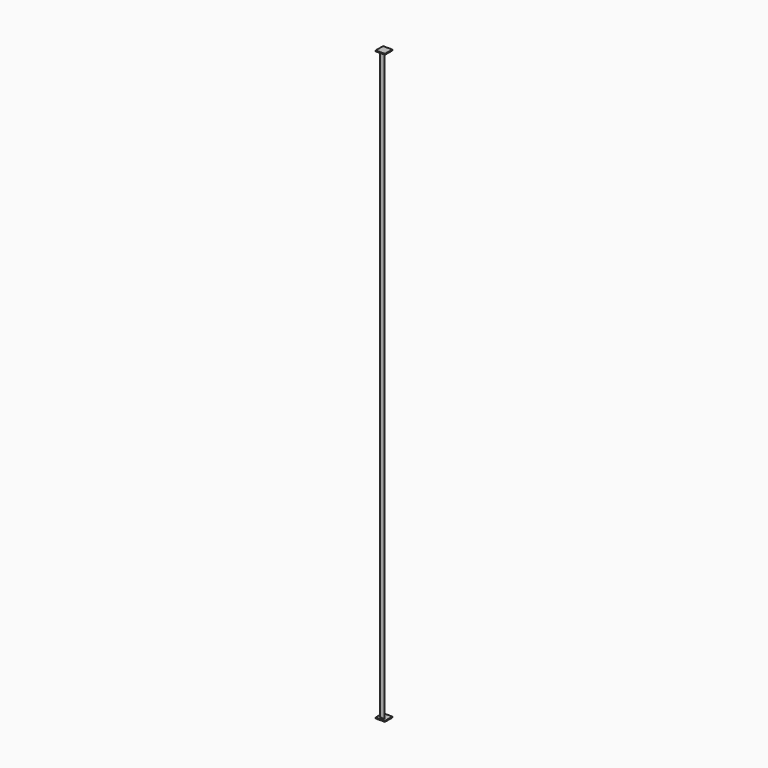
from build123d import *

# Parameters (mm, degrees)
F1_DEPTH = 1894
F2_R     = 2
F3_R     = 1.99999
F4_W     = 30
F4_H     = 30
F5_DEPTH = 3
F6_W     = 30
F6_H     = 30
F7_DEPTH = 3


# Not quite as in the source:
# - a fillet or chamfer is up to 0.001 mm smaller than in the source, because OpenCascade refuses the exact size


with BuildPart() as f1:
    # F0 (on Top) → F1 (new body)
    with BuildSketch(Plane.XY):
        Polygon((0, 15), (0, 0), (15, 0), (15, 2), (2, 2), (2, 15), align=None)
    extrude(amount=F1_DEPTH)

    # F2
    f2_edges = [f1.edges().sort_by_distance(p)[0] for p in [
        (2, 2, 947),
    ]]
    fillet(f2_edges, radius=F2_R)

    # F3 (radius 2 in the source; OpenCascade refuses exactly that, so slightly less here)
    f3_edges = [f1.edges().sort_by_distance(p)[0] for p in [
        (2, 15, 947),
        (15, 2, 947),
    ]]
    fillet(f3_edges, radius=F3_R)

    # F4 (on face) → F5 (join)
    with BuildSketch(Plane.XY.offset(1894)):
        with Locations((7.5, 7.5)):
            Rectangle(F4_W, F4_H)
    extrude(amount=F5_DEPTH)

    # F6 (on face) → F7 (join)
    with BuildSketch(Plane(origin=(0, 0, 0), x_dir=(1, 0, 0), z_dir=(0, 0, -1))):
        with Locations((7.5, -7.5)):
            Rectangle(F6_W, F6_H)
    extrude(amount=F7_DEPTH)


solid = f1.part
